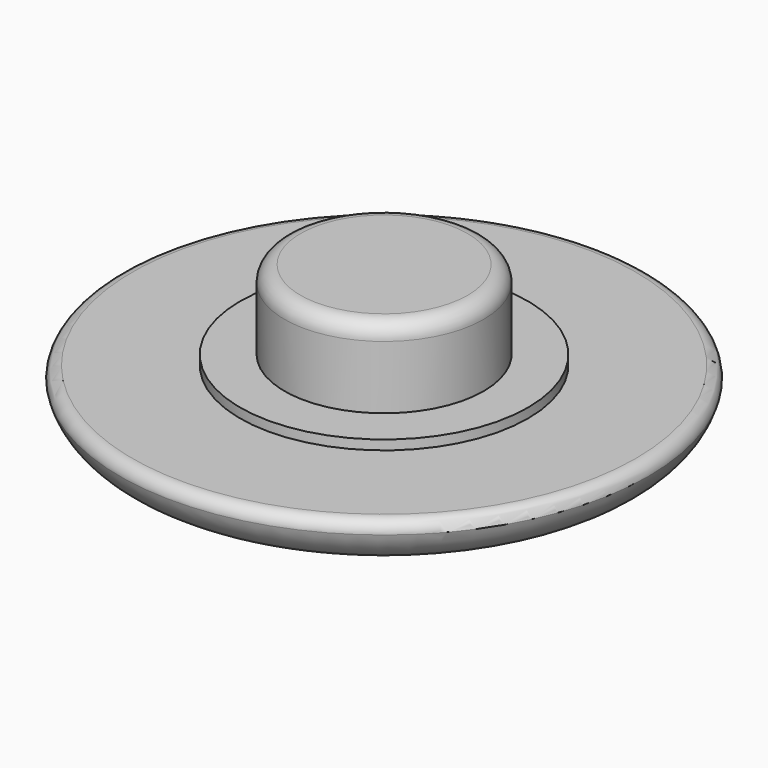
from build123d import *

# Parameters (mm, degrees)
F0_R     = 11
F0_R_2   = 6
F0_R_3   = 4.15
F1_DEPTH = 2
F2_DEPTH = 5.7
F3_R     = 0.5
F5_DEPTH = 2.4
F6_R     = 9
F6_R_2   = 8.5
F6_R_3   = 8
F6_R_4   = 7
F6_R_5   = 6.5
F6_R_6   = 6
F6_R_7   = 5
F6_R_8   = 4.5
F6_R_9   = 4
F6_R_10  = 3
F6_R_11  = 2.5
F6_R_12  = 2
F6_R_13  = 1
F6_R_14  = 0.5
F7_DEPTH = 1
F8_R     = 0.49999
F9_R     = 0.49999
F10_R    = 0.6666666667


# Not quite as in the source:
# - a fillet or chamfer that OpenCascade refuses, or shapes differently, is made with other operations: its cross-section is extruded or revolved along the edge and cut away or added
# - a fillet or chamfer is up to 0.001 mm smaller than in the source, because OpenCascade refuses the exact size


with BuildPart() as f1:
    # F0 (on Top) → F1 (new body)
    with BuildSketch(Plane.XY):
        Circle(F0_R)
        Circle(F0_R_2, mode=Mode.SUBTRACT)
        Circle(F0_R_2)
        Circle(F0_R_3, mode=Mode.SUBTRACT)
        Circle(F0_R_3)
    extrude(amount=F1_DEPTH)

    # F0 (on Top) → F2 (join)
    with BuildSketch(Plane.XY):
        Circle(F0_R_3)
    extrude(amount=F2_DEPTH)

    # F3
    f3_edges = [f1.edges().sort_by_distance(p)[0] for p in [
        (-11, 0, 2),
    ]]
    fillet(f3_edges, radius=F3_R)

    # F4: fillet of radius 2 on 1 edges, made by hand

    # F4_s1 → F4_t2 (revolve, cut)
    with BuildSketch(Plane.XZ):
        with BuildLine():
            ThreePointArc((11, 1.5), (10.2882531983, 0.4188611699), (9.0635083269, 0))
            Line((9.0635083269, 0), (9.0635083269, -0.04))
            Line((9.0635083269, -0.04), (11, -0.04))
            Line((11, -0.04), (11.04, 0))
            ThreePointArc((11.04, 0), (11.04, 0.75), (11.0387298335, 1.49))
            Line((11.0387298335, 1.49), (11, 1.5))
        make_face()
    revolve(axis=Axis((0, 0, 0), (0, 0, 1)), mode=Mode.SUBTRACT)

    # F0 (on Top) → F5 (join)
    with BuildSketch(Plane.XY):
        Circle(F0_R_2)
        Circle(F0_R_3, mode=Mode.SUBTRACT)
    extrude(amount=F5_DEPTH)

    # F6 (on Top) → F7 (cut)
    with BuildSketch(Plane.XY):
        Circle(F6_R)
        Circle(F6_R_2, mode=Mode.SUBTRACT)
        Circle(F6_R_2)
        Circle(F6_R_3, mode=Mode.SUBTRACT)
        Circle(F6_R_4)
        Circle(F6_R_5, mode=Mode.SUBTRACT)
        Circle(F6_R_5)
        Circle(F6_R_6, mode=Mode.SUBTRACT)
        Circle(F6_R_7)
        Circle(F6_R_8, mode=Mode.SUBTRACT)
        Circle(F6_R_8)
        Circle(F6_R_9, mode=Mode.SUBTRACT)
        Circle(F6_R_10)
        Circle(F6_R_11, mode=Mode.SUBTRACT)
        Circle(F6_R_11)
        Circle(F6_R_12, mode=Mode.SUBTRACT)
        Circle(F6_R_13)
        Circle(F6_R_14, mode=Mode.SUBTRACT)
        Circle(F6_R_14)
    extrude(amount=F7_DEPTH, mode=Mode.SUBTRACT)

    # F8 (radius 0.5 in the source; OpenCascade refuses exactly that, so slightly less here)
    f8_edges = [f1.edges().sort_by_distance(p)[0] for p in [
        (-1, 0, 1),
        (-2, 0, 1),
        (-3, 0, 1),
        (-4, 0, 1),
        (-5, 0, 1),
        (-6, 0, 1),
        (-7, 0, 1),
        (-9, 0, 1),
        (-8, 0, 1),
    ]]
    fillet(f8_edges, radius=F8_R)

    # F9 (radius 0.5 in the source; OpenCascade refuses exactly that, so slightly less here)
    f9_edges = [f1.edges().sort_by_distance(p)[0] for p in [
        (-2, 0, 0),
        (-1, 0, 0),
        (-4, 0, 0),
        (-3, 0, 0),
        (-9.063508, 0, 0),
        (-9, 0, 0),
        (-8, 0, 0),
        (-7, 0, 0),
        (-6, 0, 0),
        (-5, 0, 0),
    ]]
    fillet(f9_edges, radius=F9_R)

    # F10
    f10_edges = [f1.edges().sort_by_distance(p)[0] for p in [
        (-4.15, 0, 5.7),
    ]]
    fillet(f10_edges, radius=F10_R)


solid = f1.part
